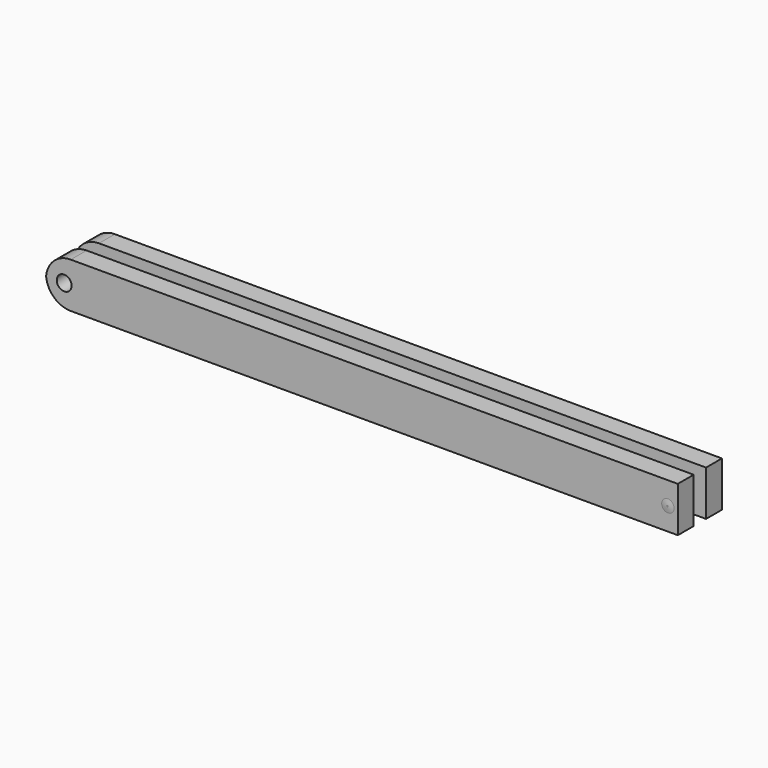
from build123d import *

# Parameters (mm, degrees)
F0_W        = 129.5146
F0_H        = 11.303
F1_DEPTH    = 9.271
F2_W        = 206.3660303733
F2_H        = 3.175
F3_DEPTH    = 7.5438
F4_W        = 3.7084
F4_H        = 3.175
F5_DEPTH    = 25.4
F6_W        = 16.3322
F6_H        = 3.175
F7_DEPTH    = 25.4
F8_T1_DEPTH = 29.464
F8_T3_DEPTH = 29.464
F9_R        = 1.524
F10_DEPTH   = 25.4
F12_DEPTH   = 0.127


# Not quite as in the source:
# - a fillet or chamfer that OpenCascade refuses, or shapes differently, is made with other operations: its cross-section is extruded or revolved along the edge and cut away or added


with BuildPart() as f1:
    # F0 (on Top) → F1 (new body)
    with BuildSketch(Plane.XY):
        Rectangle(F0_W, F0_H)
    extrude(amount=F1_DEPTH)

    # F2 (on face) → F3 (cut)
    with BuildSketch(Plane.XY.offset(9.271)):
        Rectangle(F2_W, F2_H)
    extrude(amount=-F3_DEPTH, mode=Mode.SUBTRACT)

    # F4 (on face) → F5 (cut)
    with BuildSketch(Plane.XY.offset(1.7272)):
        with Locations((62.9031, 0)):
            Rectangle(F4_W, F4_H)
    extrude(amount=-F5_DEPTH, mode=Mode.SUBTRACT)

    # F6 (on face) → F7 (cut)
    with BuildSketch(Plane.XY.offset(1.7272)):
        with Locations((-56.5912, 0)):
            Rectangle(F6_W, F6_H)
    extrude(amount=-F7_DEPTH, mode=Mode.SUBTRACT)

    # F8: fillet of radius 5.08 on 4 edges, made by hand

    # F8_s2 → F8_t1 (cut)
    with BuildSketch(Plane.XZ.offset(-11.1125)):
        with BuildLine():
            ThreePointArc((-64.7573, 4.191), (-63.2694024484, 7.7831024484), (-59.6773, 9.271))
            Line((-59.6773, 9.271), (-64.7573, 9.271))
            Line((-64.7573, 9.271), (-64.7573, 4.191))
        make_face()
        with BuildLine():
            ThreePointArc((-64.7573, 5.08), (-63.2694024484, 1.4878975516), (-59.6773, 0))
            Line((-59.6773, 0), (-64.7573, 0))
            Line((-64.7573, 0), (-64.7573, 5.08))
        make_face()
    extrude(amount=F8_T1_DEPTH, mode=Mode.SUBTRACT)

    # F8_s4 → F8_t3 (cut)
    with BuildSketch(Plane.XZ.offset(-18.3515)):
        with BuildLine():
            ThreePointArc((-59.6773, 9.271), (-63.2694024484, 7.7831024484), (-64.7573, 4.191))
            Line((-64.7573, 4.191), (-64.7573, 9.271))
            Line((-64.7573, 9.271), (-59.6773, 9.271))
        make_face()
        with BuildLine():
            ThreePointArc((-64.7573, 5.08), (-63.2694024484, 1.4878975516), (-59.6773, 0))
            Line((-59.6773, 0), (-64.7573, 0))
            Line((-64.7573, 0), (-64.7573, 5.08))
        make_face()
    extrude(amount=F8_T3_DEPTH, mode=Mode.SUBTRACT)

    # F9 (on face) → F10 (cut)
    with BuildSketch(Plane.XZ.offset(5.6515)):
        with Locations((-61.0294157593, 4.6167229302)):
            Circle(F9_R)
    extrude(amount=-F10_DEPTH, mode=Mode.SUBTRACT)

    # F11 (on face) → F12 (join)
    with BuildSketch(Plane.XZ.offset(5.6515)):
        with BuildLine():
            Line((61.4553, 4.6355), (63.9953, 4.6355))
            ThreePointArc((63.9953, 4.6355), (62.7253, 5.9055), (61.4553, 4.6355))
        make_face()
        with BuildLine():
            ThreePointArc((61.4553, 4.6355), (62.7253, 3.3655), (63.9953, 4.6355))
            Line((63.9953, 4.6355), (61.4553, 4.6355))
        make_face()
    extrude(amount=F12_DEPTH)

    # F13: fillet of radius 5.08 on 1 edges, made by hand

    # F13_s1 → F13_t2 (revolve, cut)
    with BuildSketch(Plane.XY.offset(4.6355)):
        with BuildLine():
            ThreePointArc((61.4553, -5.6515), (62.0161394247, -5.7466501562), (62.584100691, -5.7785))
            Line((62.584100691, -5.7785), (61.4553, -5.7785))
            Line((61.4553, -5.7785), (61.4553, -5.6515))
        make_face()
    revolve(axis=Axis((62.7253, -5.7785, 4.6355), (0, -1, 0)), mode=Mode.SUBTRACT)

    # F14: F1 across plane


with BuildPart() as f1_1:
    add(f1.part)
    add(f1.part.mirror(Plane.XZ))


solid = f1_1.part
